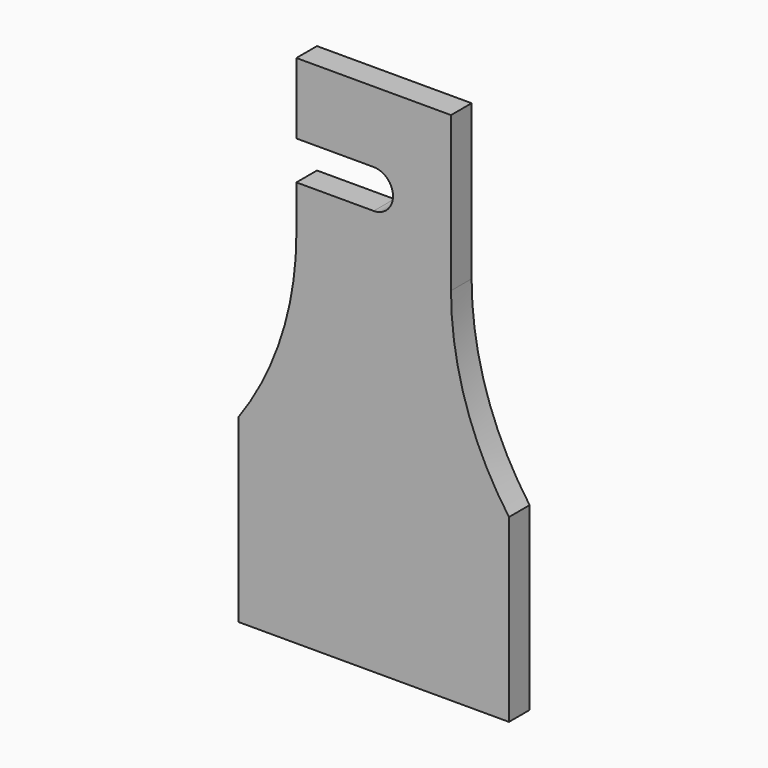
from build123d import *

# Parameters (mm, degrees)
F0_W     = 133.35
F0_H     = 254
F1_DEPTH = 12.7
F3_DEPTH = 294
F5_DEPTH = 12.701


# Not quite as in the source:
# - an extrude ends at something that could not be found from the text; its depth is read off the source's solid
# - a pattern or mirror of a feature is missing from the dataset's text; its kind, count and spacing are read off the source's solid


with BuildPart() as f1:
    # F0 (on Front) → F1 (new body)
    with BuildSketch(Plane.XZ):
        Rectangle(F0_W, F0_H)
    extrude(amount=F1_DEPTH)

    # F0 (on Front) + F2 (on face) → F3 (cut, through all)
    with BuildSketch(Plane.XZ):
        Rectangle(F0_W, F0_H)
    with BuildSketch(Plane.XZ.offset(12.7)):
        with BuildLine():
            Line((-66.675, 73.025), (0, 73.025))
            ThreePointArc((0, 73.025), (9.525, 82.55), (0, 92.075))
            Line((0, 92.075), (-66.675, 92.075))
            Line((-66.675, 92.075), (-66.675, 73.025))
        make_face()
    extrude(amount=-F3_DEPTH, mode=Mode.SUBTRACT)

    # F4 (on face) → F5 (cut, through all)
    with BuildSketch(Plane.XZ.offset(12.7)):
        with BuildLine():
            Line((66.675, 127), (38.1, 127))
            Line((38.1, 127), (38.1, 50.8))
            ThreePointArc((38.1, 50.8), (45.4193088889, 4.1102242857), (66.675, -38.1))
            Line((66.675, -38.1), (66.675, 127))
        make_face()
    f5 = extrude(amount=-F5_DEPTH, mode=Mode.SUBTRACT)

    # F5_copies: F5 across plane
    add(f5.mirror(Plane(origin=(0, 0, 0), x_dir=(0, 0, -1), z_dir=(-1, 0, 0))), mode=Mode.SUBTRACT)


solid = f1.part
